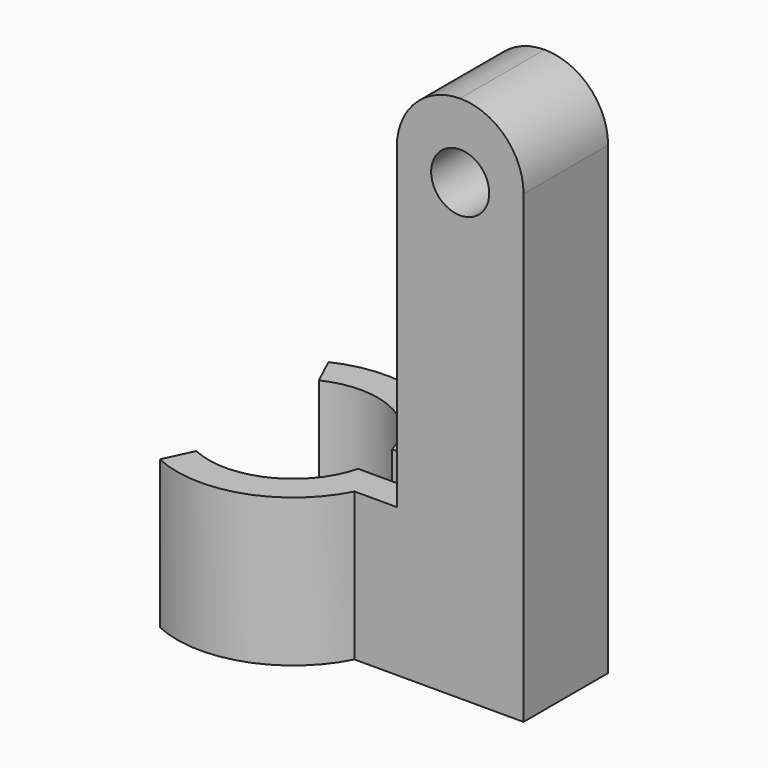
from build123d import *

# Parameters (mm, degrees)
F1_DEPTH = 7
F0_W     = 6
F0_H     = 5
F2_DEPTH = 25
F3_R     = 1.3748922144
F4_DEPTH = 25
F5_R     = 2.99999
F7_DEPTH = 25


# Not quite as in the source:
# - a fillet or chamfer is up to 0.001 mm smaller than in the source, because OpenCascade refuses the exact size


with BuildPart() as f1:
    # F0 (on Top) → F1 (new body)
    with BuildSketch(Plane.XY):
        with BuildLine():
            ThreePointArc((-1.690473047, 3.6252311481), (2.1491984334, 3.3735657833), (4, 0))
            ThreePointArc((4, 0), (2.1491984334, -3.3735657833), (-1.690473047, -3.6252311481))
            Line((-1.690473047, -3.6252311481), (-2.3244004396, -4.9846928287))
            ThreePointArc((-2.3244004396, -4.9846928287), (1.789005011, -5.2009096388), (4.8989794856, -2.5))
            ThreePointArc((4.8989794856, -2.5), (5.3476343915, -1.2856151892), (5.5, 0))
            ThreePointArc((5.5, 0), (5.3476343915, 1.2856151892), (4.8989794856, 2.5))
            ThreePointArc((4.8989794856, 2.5), (1.789005011, 5.2009096388), (-2.3244004396, 4.9846928287))
            Line((-2.3244004396, 4.9846928287), (-1.690473047, 3.6252311481))
        make_face()
        with BuildLine():
            Line((6.8989794856, 2.5), (4.8989794856, 2.5))
            ThreePointArc((4.8989794856, 2.5), (5.3476343915, 1.2856151892), (5.5, 0))
            ThreePointArc((5.5, 0), (5.3476343915, -1.2856151892), (4.8989794856, -2.5))
            Line((4.8989794856, -2.5), (6.8989794856, -2.5))
            Line((6.8989794856, -2.5), (6.8989794856, 2.5))
        make_face()
    extrude(amount=F1_DEPTH)

    # F0 (on Top) → F2 (join)
    with BuildSketch(Plane.XY):
        with Locations((9.8989794856, 0)):
            Rectangle(F0_W, F0_H)
    extrude(amount=F2_DEPTH)

    # F3 (on face) → F4 (cut)
    with BuildSketch(Plane.XZ.offset(2.5)):
        with Locations((9.8989794856, 21.5)):
            Circle(F3_R)
    extrude(amount=-F4_DEPTH, mode=Mode.SUBTRACT)

    # F5 (radius 3 in the source; OpenCascade refuses exactly that, so slightly less here)
    f5_edges = [f1.edges().sort_by_distance(p)[0] for p in [
        (12.898979, 0, 25),
        (6.898979, 0, 25),
    ]]
    fillet(f5_edges, radius=F5_R)

    # F6 (on face) → F7 (cut)
    with BuildSketch(Plane.XY.offset(7)):
        with BuildLine():
            Line((3.8729833462, -1), (6.8989794856, -1))
            Line((6.8989794856, -1), (6.8989794856, 1))
            Line((6.8989794856, 1), (3.8729833462, 1))
            ThreePointArc((3.8729833462, 1), (4, 0), (3.8729833462, -1))
        make_face()
    extrude(amount=-F7_DEPTH, mode=Mode.SUBTRACT)


solid = f1.part
